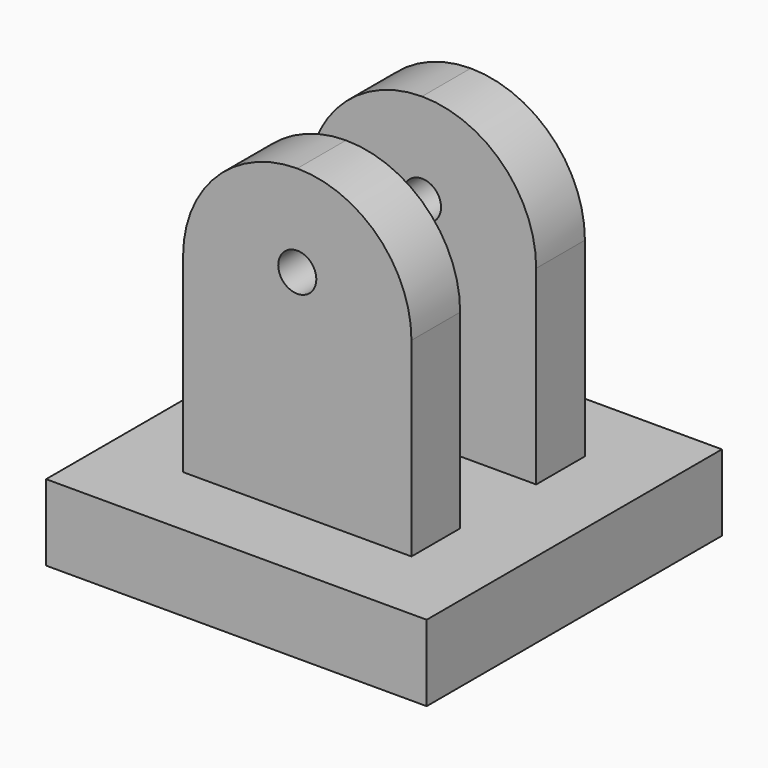
from build123d import *

# Parameters (mm, degrees)
F0_W     = 50
F0_H     = 48.4855457247
F1_DEPTH = 10
F2_W     = 30
F2_H     = 8
F4_DEPTH = 40
F3_W     = 30
F3_H     = 8
F5_DEPTH = 40
F7_D     = 5
F8_R     = 14.99999


# Not quite as in the source:
# - a fillet or chamfer is up to 0.001 mm smaller than in the source, because OpenCascade refuses the exact size


with BuildPart() as f1:
    # F0 (on Top) → F1 (new body)
    with BuildSketch(Plane.XY):
        with Locations((-4.2565334588, 1.5670973808)):
            Rectangle(F0_W, F0_H)
    extrude(amount=F1_DEPTH)

    # F2 (on face) → F4 (join)
    with BuildSketch(Plane.XY.offset(10)):
        with Locations((-4.2565334588, 11.8098702431)):
            Rectangle(F2_W, F2_H)
    extrude(amount=F4_DEPTH)

    # F3 (on face) → F5 (join)
    with BuildSketch(Plane.XY.offset(10)):
        with Locations((-4.2565334588, -8.6756754816)):
            Rectangle(F3_W, F3_H)
    extrude(amount=F5_DEPTH)

    # F7 (through all)
    with Locations(Plane.XZ.offset(12.6756754816)):
        with Locations((-4.2565334588, 38)):
            Hole(F7_D / 2)

    # F8 (radius 15 in the source; OpenCascade refuses exactly that, so slightly less here)
    f8_edges = [f1.edges().sort_by_distance(p)[0] for p in [
        (10.743467, -8.675675, 50),
        (-19.256533, -8.675675, 50),
        (10.743467, 11.80987, 50),
        (-19.256533, 11.80987, 50),
    ]]
    fillet(f8_edges, radius=F8_R)


solid = f1.part
